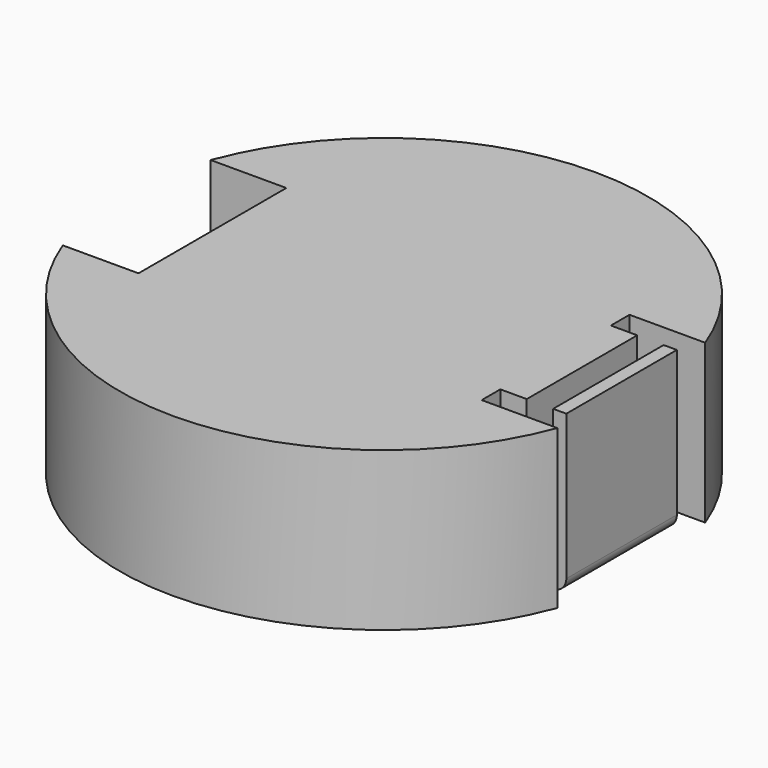
from build123d import *

# Parameters (mm, degrees)
F0_R         = 20
F1_DEPTH     = 12
F3_D         = 3.1
F3_DEPTH     = 8
F3_TIP       = 0.9313339595
F5_DEPTH     = 12.001
F6_W         = 5
F6_H         = 10.46546828
F7_DEPTH     = 12
F8_W         = 2
F8_H         = 10.46546828
F9_DEPTH     = 11
F10_W        = 1
F10_H        = 10.46546828
F11_DEPTH    = 5
F12_T1_DEPTH = 10.46546828
F12_T3_DEPTH = 10.46546828


# Not quite as in the source:
# - a fillet or chamfer that OpenCascade refuses, or shapes differently, is made with other operations: its cross-section is extruded or revolved along the edge and cut away or added


with BuildPart() as f1:
    # F0 (on Top) → F1 (new body)
    with BuildSketch(Plane.XY):
        Circle(F0_R)
    extrude(amount=F1_DEPTH)

    # F3
    with Locations(Plane(origin=(0, 0, 0), x_dir=(1, 0, 0), z_dir=(0, 0, -1))):
        with Locations((-10.9601551084, 10.9601551084), (-10.9601551084, -10.9601551084), (10.9601551084, -10.9601551084), (10.9601551084, 10.9601551084)):
            Hole(F3_D / 2, depth=F3_DEPTH)
            with Locations((0, 0, -(F3_DEPTH + F3_TIP / 2))):  # 118° drill point
                Cone(0, F3_D / 2, F3_TIP, mode=Mode.SUBTRACT)

    # F4 (on face) → F5 (intersect, through all)
    with BuildSketch(Plane.XY.offset(12)):
        with BuildLine():
            Line((13, -7), (13, 7))
            Line((13, 7), (18.7349939952, 7))
            ThreePointArc((18.7349939952, 7), (0, 20), (-18.7349939952, 7))
            Line((-18.7349939952, 7), (-13, 7))
            Line((-13, 7), (-13, -7))
            Line((-13, -7), (-18.7349939952, -7))
            ThreePointArc((-18.7349939952, -7), (0, -20), (18.7349939952, -7))
            Line((18.7349939952, -7), (13, -7))
        make_face()
    extrude(amount=-F5_DEPTH, mode=Mode.INTERSECT)

    # F6 (on Top) → F7 (join)
    with BuildSketch(Plane.XY):
        with Locations((15.5, 0)):
            Rectangle(F6_W, F6_H)
    extrude(amount=F7_DEPTH)

    # F8 (on face) → F9 (cut)
    with BuildSketch(Plane.XY.offset(12)):
        with Locations((16, 0)):
            Rectangle(F8_W, F8_H)
    extrude(amount=-F9_DEPTH, mode=Mode.SUBTRACT)

    # F10 (on Top) → F11 (cut)
    with BuildSketch(Plane.XY):
        with Locations((13.5, 0)):
            Rectangle(F10_W, F10_H)
    extrude(amount=F11_DEPTH, mode=Mode.SUBTRACT)

    # F12: fillet of radius 1 on 6 edges, made by hand

    # F12_s2 → F12_t1 (join)
    with BuildSketch(Plane.XZ.offset(-5.23273414)):
        with BuildLine():
            ThreePointArc((15, 2), (15.2928932188, 1.2928932188), (16, 1))
            Line((16, 1), (15, 1))
            Line((15, 1), (15, 2))
        make_face()
        with BuildLine():
            ThreePointArc((16, 1), (16.7071067812, 1.2928932188), (17, 2))
            Line((17, 2), (17, 1))
            Line((17, 1), (16, 1))
        make_face()
        with BuildLine():
            ThreePointArc((14, 4), (13.7071067812, 4.7071067812), (13, 5))
            Line((13, 5), (14, 5))
            Line((14, 5), (14, 4))
        make_face()
        with BuildLine():
            ThreePointArc((13, 4), (13.2928932188, 4.7071067812), (14, 5))
            Line((14, 5), (13, 5))
            Line((13, 5), (13, 4))
        make_face()
    extrude(amount=F12_T1_DEPTH)

    # F12_s4 → F12_t3 (cut)
    with BuildSketch(Plane.XZ.offset(-5.23273414)):
        with BuildLine():
            ThreePointArc((18, 1), (17.7071067812, 0.2928932188), (17, 0))
            Line((17, 0), (18, 0))
            Line((18, 0), (18, 1))
        make_face()
        with BuildLine():
            ThreePointArc((14, 1), (14.2928932188, 0.2928932188), (15, 0))
            Line((15, 0), (14, 0))
            Line((14, 0), (14, 1))
        make_face()
    extrude(amount=F12_T3_DEPTH, mode=Mode.SUBTRACT)


solid = f1.part
